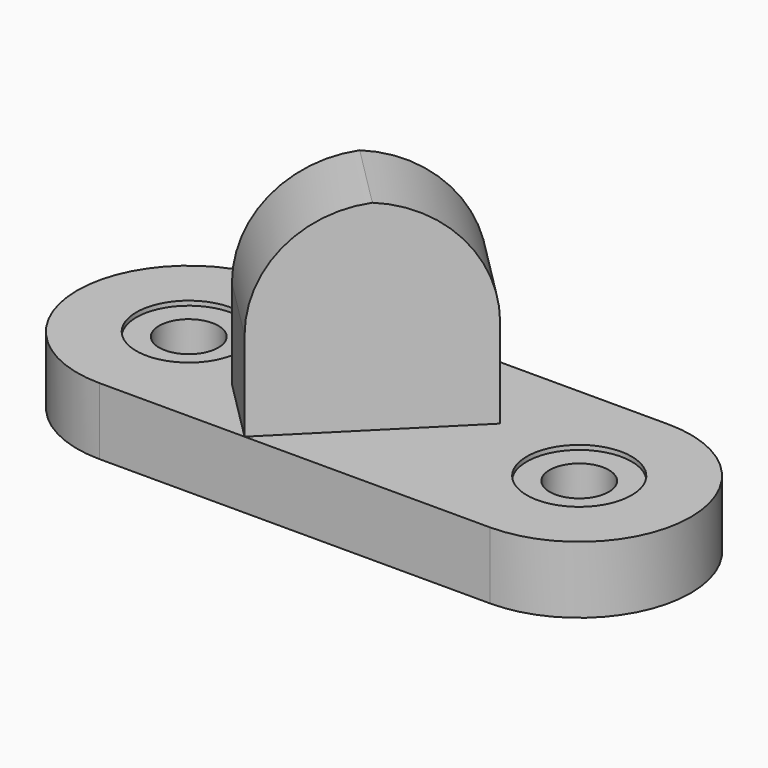
from build123d import *

# Parameters (mm, degrees)
F0_R        = 11.938
F1_DEPTH    = 15.24
F0_R_2      = 6.7437
F2_DEPTH    = 14.224
F5_DEPTH    = 45.72
F6_T1_DEPTH = 147.32
F6_T3_DEPTH = 147.32


# Not quite as in the source:
# - a fillet or chamfer that OpenCascade refuses, or shapes differently, is made with other operations: its cross-section is extruded or revolved along the edge and cut away or added


with BuildPart() as f1:
    # F0 (on Top) → F1 (new body)
    with BuildSketch(Plane.XY):
        with BuildLine():
            ThreePointArc((44.45, -25.4), (69.85, 0), (44.45, 25.4))
            Line((44.45, 25.4), (-44.45, 25.4))
            ThreePointArc((-44.45, 25.4), (-69.85, 0), (-44.45, -25.4))
            Line((-44.45, -25.4), (44.45, -25.4))
        make_face()
        with Locations((-44.45, 0)):
            Circle(F0_R, mode=Mode.SUBTRACT)
        with Locations((44.45, 0)):
            Circle(F0_R, mode=Mode.SUBTRACT)
    extrude(amount=F1_DEPTH)

    # F0 (on Top) → F2 (join)
    with BuildSketch(Plane.XY):
        with Locations((-44.45, 0)):
            Circle(F0_R)
        with Locations((-44.45, 0)):
            Circle(F0_R_2, mode=Mode.SUBTRACT)
        with Locations((44.45, 0)):
            Circle(F0_R)
        with Locations((44.45, 0)):
            Circle(F0_R_2, mode=Mode.SUBTRACT)
    extrude(amount=F2_DEPTH)

    # F4 (on face) → F5 (join)
    with BuildSketch(Plane.XY.offset(15.24)):
        Polygon((-25.7984097937, -11.0315902063), (-11.43, -25.4), (20.8989220358, 6.9289220358), (6.5305122421, 21.2973318296), align=None)
    extrude(amount=F5_DEPTH)

    # F6: fillet of radius 25.4 on 2 edges, made by hand

    # F6_s2 → F6_t1 (cut)
    with BuildSketch(Plane(origin=(-52.2846903991, 52.2846903991, 0), x_dir=(0, 0, 1), z_dir=(0.7071067812, -0.7071067812, 0))):
        with BuildLine():
            ThreePointArc((35.56, 26.0427427511), (53.5205122421, 18.6032549932), (60.96, 0.6427427511))
            Line((60.96, 0.6427427511), (60.96, 26.0427427511))
            Line((60.96, 26.0427427511), (35.56, 26.0427427511))
        make_face()
    extrude(amount=F6_T1_DEPTH, mode=Mode.SUBTRACT)

    # F6_s4 → F6_t3 (cut)
    with BuildSketch(Plane(origin=(51.8862806053, -51.8862806053, 0), x_dir=(0, 0, 1), z_dir=(-0.7071067812, 0.7071067812, 0))):
        with BuildLine():
            ThreePointArc((35.56, 19.6772572489), (53.5205122421, 12.237769491), (60.96, -5.7227427511))
            Line((60.96, -5.7227427511), (60.96, 19.6772572489))
            Line((60.96, 19.6772572489), (35.56, 19.6772572489))
        make_face()
    extrude(amount=F6_T3_DEPTH, mode=Mode.SUBTRACT)


solid = f1.part
